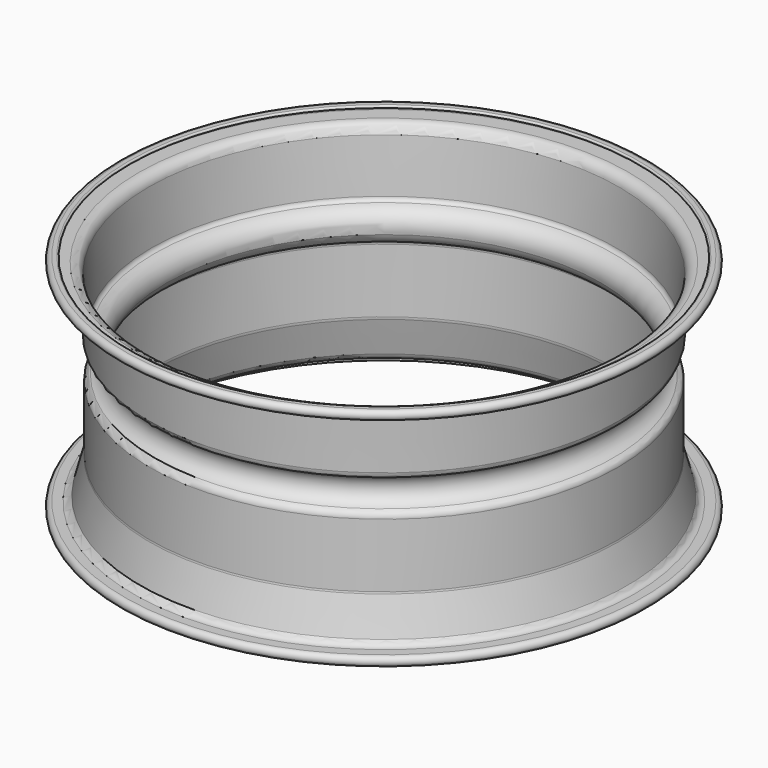
from build123d import *


# Not quite as in the source:
# - ends of sketch curves that miss each other by under 0.0002 mm in the source are joined


with BuildPart() as f1:
    # F0 (on Front) → F1 (revolve)
    with BuildSketch(Plane.XZ):
        with BuildLine():
            Line((-119.9645374891, -19.0556111847), (-126.1162052209, -19.0556111847))
            ThreePointArc((-126.1162052209, -19.0556111847), (-129.365444403, -22.5181057669), (-125.9725242853, -25.8399301254))
            Line((-125.9725242853, -25.8399301254), (-124.8474305217, -25.8399301254))
            ThreePointArc((-124.8474305217, -25.8399301254), (-123.8474305217, -24.8399301254), (-124.8474305217, -23.8399301254))
            Line((-124.8474305217, -23.8399301254), (-125.9725242853, -23.8399301254))
            ThreePointArc((-125.9725242853, -23.8399301254), (-127.510217073, -22.5234139406), (-126.1162052209, -21.0556111847))
            Line((-126.1162052209, -21.0556111847), (-119.9645374891, -21.0556111847))
            ThreePointArc((-119.9645374891, -21.0556111847), (-115.6950439438, -19.6028109167), (-113.1977565033, -15.8474468608))
            Line((-113.1977565033, -15.8474468608), (-106.6701284805, 8.8038254501))
            ThreePointArc((-106.6701284805, 8.8038254501), (-106.4954590811, 9.6921864172), (-106.4369094663, 10.5956611262))
            Line((-106.4369094663, 10.5956611262), (-106.4369094663, 55.3331610558))
            ThreePointArc((-106.4369094663, 55.3331610558), (-105.8788017228, 57.0759066503), (-104.4121346614, 58.1702257041))
            ThreePointArc((-104.4121346614, 58.1702257041), (-99.4693510462, 61.3422466364), (-96.5444093761, 66.4351380438))
            ThreePointArc((-96.5444093761, 66.4351380438), (-97.6011497884, 75.8685945768), (-105.02732781, 81.7811813584))
            ThreePointArc((-105.02732781, 81.7811813584), (-106.5489920048, 82.7976382138), (-107.197096774, 84.5089554458))
            Line((-107.197096774, 84.5089554458), (-109.1252628864, 121.4850969167))
            ThreePointArc((-109.1252628864, 121.4850969167), (-109.1254842953, 121.4893183303), (-109.125703155, 121.4935398784))
            ThreePointArc((-109.125703155, 121.4935398784), (-111.2970609996, 126.2060037188), (-116.1162052209, 128.1290116))
            Line((-116.1162052209, 128.1290116), (-126.2854278027, 128.1290116))
            ThreePointArc((-126.2854278027, 128.1290116), (-127.5380970484, 129.4662744669), (-126.1219410502, 130.6290102076))
            Line((-126.1219410502, 130.6290102076), (-123.4164699041, 130.6290102076))
            ThreePointArc((-123.4164699041, 130.6290102076), (-122.4164699041, 131.6290102076), (-123.4164699041, 132.6290102076))
            Line((-123.4164699041, 132.6290102076), (-126.1192136336, 132.6290102076))
            ThreePointArc((-126.1192136336, 132.6290102076), (-129.3662048728, 129.3775073935), (-126.1162052209, 126.1290116))
            Line((-126.1162052209, 126.1290116), (-116.1162052209, 126.1290116))
            ThreePointArc((-116.1162052209, 126.1290116), (-112.6739593486, 124.755434542), (-111.1229894595, 121.3893889417))
            Line((-111.1229894595, 121.3893889417), (-109.1943830786, 84.4048045091))
            ThreePointArc((-109.1943830786, 84.4048045091), (-108.1142084632, 81.5526091224), (-105.5781014718, 79.8585143635))
            ThreePointArc((-105.5781014718, 79.8585143635), (-98.0593686139, 70.1492420154), (-105.0622847915, 60.0616021363))
            ThreePointArc((-105.0622847915, 60.0616021363), (-107.5067298939, 58.2377370467), (-108.4369094663, 55.3331610558))
            Line((-108.4369094663, 55.3331610558), (-108.4369094663, 10.5956611262))
            ThreePointArc((-108.4369094663, 10.5956611262), (-108.4787306197, 9.9503220484), (-108.6034944764, 9.3157785004))
            Line((-108.6034944764, 9.3157785004), (-115.1311224993, -15.3354938105))
            ThreePointArc((-115.1311224993, -15.3354938105), (-116.9148992425, -18.0178967075), (-119.9645374891, -19.0556111847))
        make_face()
    revolve(axis=Axis((55.6337947791, 0, 51.8589288074), (0, 0, -1)))


solid = f1.part
